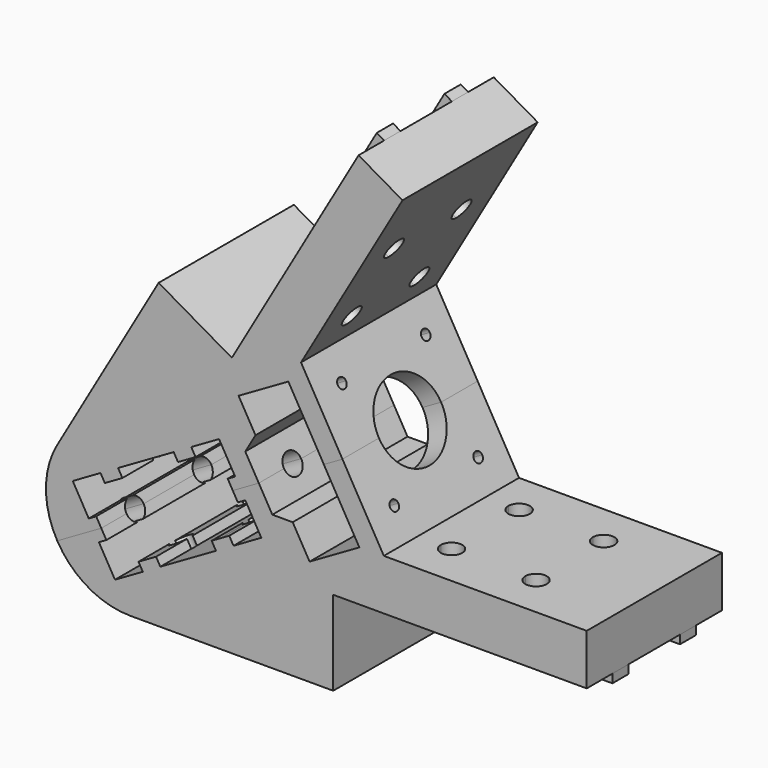
from build123d import *
from build123d import SkipClean  # not in build123d's __all__

# Parameters (mm, degrees)
F1_DEPTH  = 50
F3_DEPTH  = 50
F4_W      = 6
F4_H      = 75
F5_DEPTH  = 2.54
F7_DEPTH  = 78.4977147554
F8_W      = 53.81
F8_H      = 3.175
F13_W     = 6.35
F13_H     = 6.35
F17_DEPTH = 6.35
F19_DEPTH = 50.0010001
F22_W     = 3.175
F22_H     = 8.0837567297
F22_H_2   = 12.5575134595
F22_H_3   = 6.35


with BuildPart() as f1:
    # F0 (on Front) → F1 (new body)
    with BuildSketch(Plane.XZ):
        with BuildLine():
            Line((80.4903810568, 109.4134295109), (67.5, 116.9134295109))
            Line((67.5, 116.9134295109), (30, 51.9615242271))
            Line((30, 51.9615242271), (8.3493649054, 64.4615242271))
            Line((8.3493649054, 64.4615242271), (-21.6506350946, 12.5))
            ThreePointArc((-21.6506350946, 12.5), (-25, 0), (-21.6506350946, -12.5))
            Line((-21.6506350946, -12.5), (-10.8253175473, -6.25))
            Line((-10.8253175473, -6.25), (-17.0753175473, 4.5753175473))
            Line((-17.0753175473, 4.5753175473), (-6.25, 10.8253175473))
            Line((-6.25, 10.8253175473), (26.2259526419, 29.5753175473))
            Line((26.2259526419, 29.5753175473), (32.4759526419, 18.75))
            Line((32.4759526419, 18.75), (37.9752139559, 21.925))
            Line((37.9752139559, 21.925), (33.9770633418, 28.85))
            Line((33.9770633418, 28.85), (46.8086730745, 51.075))
            Line((46.8086730745, 51.075), (50.4748472839, 57.425))
            Line((50.4748472839, 57.425), (80.4903810568, 109.4134295109))
        make_face()
        Polygon((62.7218898691, 36.2125), (50.4748472839, 57.425), (46.8086730745, 51.075), (57.2226285551, 33.0375), align=None)
    extrude(amount=F1_DEPTH)

    # F2 (on face) → F3 (join, through all)
    with BuildSketch(Plane(origin=(0, 0, 0), x_dir=(-1, 0, 0), z_dir=(0, 1, 0))):
        Polygon((-15.4006350946, 23.3253175473), (-17.998711306, 24.8253175473), (-19.268711306, 22.6256130217), (-16.6706350946, 21.1256130217), align=None)
        Polygon((-12.8025588833, 21.8253175473), (-15.4006350946, 23.3253175473), (-16.6706350946, 21.1256130217), (-14.0725588833, 19.6256130217), align=None)
        Polygon((-28.7762481163, 20.0780762114), (-30.9759526419, 21.3480762114), (-32.4759526419, 18.75), (-30.2762481163, 17.48), align=None)
        Polygon((10.8253175473, -6.25), (12.3253175473, -3.6519237886), (10.1256130217, -2.3819237886), (8.6256130217, -4.98), align=None)
        Polygon((6.25, 10.8253175473), (3.6519237886, 12.3253175473), (2.3819237886, 10.1256130217), (4.98, 8.6256130217), align=None)
        Polygon((8.8480762114, 9.3253175473), (6.25, 10.8253175473), (4.98, 8.6256130217), (7.5780762114, 7.1256130217), align=None)
    extrude(amount=-F3_DEPTH)

    # F4 (on face) → F5 (join)
    with BuildSketch(Plane(origin=(0, 0, 0), x_dir=(0, -1, 0), z_dir=(-0.8660254038, 0, 0.5))):
        with Locations((12.5, 97.5)):
            Rectangle(F4_W, F4_H)
        with Locations((37.5, 97.5)):
            Rectangle(F4_W, F4_H)
    extrude(amount=F5_DEPTH)

    # F6 (on face) → F7 (cut, through all)
    with BuildSketch(Plane(origin=(-2.1997045256, 0, 1.27), x_dir=(0, -1, 0), z_dir=(-0.8660254038, 0, 0.5))):
        with BuildLine():
            ThreePointArc((12.5, 88.175), (9.325, 85), (12.5, 81.825))
            Line((12.5, 81.825), (12.5, 85))
            Line((12.5, 85), (12.5, 88.175))
        make_face()
        with BuildLine():
            ThreePointArc((12.5, 113.175), (9.325, 110), (12.5, 106.825))
            Line((12.5, 106.825), (12.5, 110))
            Line((12.5, 110), (12.5, 113.175))
        make_face()
        with BuildLine():
            Line((12.5, 110), (12.5, 106.825))
            ThreePointArc((12.5, 106.825), (14.7450640303, 107.7549359697), (15.675, 110))
            ThreePointArc((15.675, 110), (14.7450640303, 112.2450640303), (12.5, 113.175))
            Line((12.5, 113.175), (12.5, 110))
        make_face()
        with BuildLine():
            Line((12.5, 85), (12.5, 81.825))
            ThreePointArc((12.5, 81.825), (14.7450640303, 82.7549359697), (15.675, 85))
            ThreePointArc((15.675, 85), (14.7450640303, 87.2450640303), (12.5, 88.175))
            Line((12.5, 88.175), (12.5, 85))
        make_face()
        with BuildLine():
            ThreePointArc((37.5, 88.175), (34.325, 85), (37.5, 81.825))
            Line((37.5, 81.825), (37.5, 85))
            Line((37.5, 85), (37.5, 88.175))
        make_face()
        with BuildLine():
            ThreePointArc((37.5, 113.175), (34.325, 110), (37.5, 106.825))
            Line((37.5, 106.825), (37.5, 110))
            Line((37.5, 110), (37.5, 113.175))
        make_face()
        with BuildLine():
            Line((37.5, 110), (37.5, 106.825))
            ThreePointArc((37.5, 106.825), (39.7450640303, 107.7549359697), (40.675, 110))
            ThreePointArc((40.675, 110), (39.7450640303, 112.2450640303), (37.5, 113.175))
            Line((37.5, 113.175), (37.5, 110))
        make_face()
        with BuildLine():
            Line((37.5, 85), (37.5, 81.825))
            ThreePointArc((37.5, 81.825), (39.7450640303, 82.7549359697), (40.675, 85))
            ThreePointArc((40.675, 85), (39.7450640303, 87.2450640303), (37.5, 88.175))
            Line((37.5, 88.175), (37.5, 85))
        make_face()
    extrude(amount=-F7_DEPTH, mode=Mode.SUBTRACT)

    # F8 (on face) → F9 (revolve, cut)
    with BuildSketch(Plane(origin=(0, 0, 0), x_dir=(0.8660254038, 0, 0.5), z_dir=(0.5, 0, -0.8660254038))):
        Polygon((-9.96, 9.325), (-9.96, 12.5), (-25, 12.5), (-25, 6.15), (-21.825, 6.15), (-21.825, 9.325), align=None)
        with Locations((16.945, 10.9125)):
            Rectangle(F8_W, F8_H)
    revolve(axis=Axis((-15.1381240582, -12.5, -8.74), (-0.8660254038, 0, -0.5)), mode=Mode.SUBTRACT)

    # F8 (on face) → F10 (revolve, cut)
    with BuildSketch(Plane(origin=(0, 0, 0), x_dir=(0.8660254038, 0, 0.5), z_dir=(0.5, 0, -0.8660254038))):
        Polygon((-21.825, 34.325), (-9.96, 34.325), (-9.96, 37.5), (-25, 37.5), (-25, 31.15), (-21.825, 31.15), align=None)
        with Locations((16.945, 35.9125)):
            Rectangle(F8_W, F8_H)
    revolve(axis=Axis((-15.1381240582, -37.5, -8.74), (-0.8660254038, 0, -0.5)), mode=Mode.SUBTRACT)

    # F13 (on face) → F14 (revolve, cut)
    with BuildSketch(Plane(origin=(21.6506350946, 0, 12.5), x_dir=(0, 1, 0), z_dir=(0.8660254038, 0, 0.5))):
        with Locations((-9.325, 46.4762701892)):
            Rectangle(F13_W, F13_H)
        Polygon((-12.5, 9.96), (-9.325, 9.96), (-9.325, 36.9512701892), (-6.15, 36.9512701892), (-6.15, 43.3012701892), (-12.5, 43.3012701892), align=None)
    revolve(axis=Axis((8.3353175473, -12.5, 35.5628065108), (-0.5, 0, 0.8660254038)), mode=Mode.SUBTRACT)

    # F13 (on face) → F15 (revolve, cut)
    with BuildSketch(Plane(origin=(21.6506350946, 0, 12.5), x_dir=(0, 1, 0), z_dir=(0.8660254038, 0, 0.5))):
        with Locations((-34.325, 46.4762701892)):
            Rectangle(F13_W, F13_H)
        Polygon((-37.5, 9.96), (-34.325, 9.96), (-34.325, 36.9512701892), (-31.15, 36.9512701892), (-31.15, 43.3012701892), (-37.5, 43.3012701892), align=None)
    revolve(axis=Axis((6.7478175473, -37.5, 38.3124371679), (-0.5, 0, 0.8660254038)), mode=Mode.SUBTRACT)

    # F16 (on face) → F17 (cut, through all)
    with BuildSketch(Plane(origin=(62.7218898691, 0, 36.2125), x_dir=(0, 1, 0), z_dir=(0.8660254038, 0, 0.5))):
        with BuildLine():
            ThreePointArc((-8, 15.5), (-9.5, 17), (-11, 15.5))
            Line((-11, 15.5), (-9.5, 15.5))
            Line((-9.5, 15.5), (-9.5, 14))
            ThreePointArc((-9.5, 14), (-8.4393398282, 14.4393398282), (-8, 15.5))
        make_face()
        with BuildLine():
            Line((-9.5, 15.5), (-11, 15.5))
            ThreePointArc((-11, 15.5), (-10.5606601718, 14.4393398282), (-9.5, 14))
            Line((-9.5, 14), (-9.5, 15.5))
        make_face()
        with BuildLine():
            ThreePointArc((-40.5, 14), (-39.4393398282, 14.4393398282), (-39, 15.5))
            Line((-39, 15.5), (-40.5, 15.5))
            Line((-40.5, 15.5), (-40.5, 14))
        make_face()
        with BuildLine():
            Line((-40.5, 15.5), (-39, 15.5))
            ThreePointArc((-39, 15.5), (-41.5606601718, 16.5606601718), (-40.5, 14))
            Line((-40.5, 14), (-40.5, 15.5))
        make_face()
        with BuildLine():
            ThreePointArc((-13.5, 0), (-25, 11.5), (-36.5, 0))
            Line((-36.5, 0), (-13.5, 0))
        make_face()
    extrude(amount=-F17_DEPTH, mode=Mode.SUBTRACT)

    # F18 (on face) → F19 (cut, through all)
    with BuildSketch(Plane.XZ.offset(50)):
        Polygon((46.7226285551, 51.2240334795), (32.0001966907, 42.7240334795), (36.9937184983, 34.075), (46.8086730745, 51.075), align=None)
    extrude(amount=-F19_DEPTH, mode=Mode.SUBTRACT)

    # F22 (on face) → F23 (revolve, cut)
    with BuildSketch(Plane(origin=(0, 0, 0), x_dir=(0, 1, 0), z_dir=(0.8660254038, 0, 0.5))):
        Polygon((-40.675, 28.8675134595), (-40.675, 36.9512701892), (-37.5, 36.9512701892), (-37.5, 41.5675134595), (-43.85, 41.5675134595), (-43.85, 28.8675134595), align=None)
        with Locations((-39.0875, 32.9093918244)):
            Rectangle(F22_W, F22_H)
        with Locations((-39.0875, 16.2387567297)):
            Rectangle(F22_W, F22_H_2)
        with Locations((-39.0875, 25.6925134595)):
            Rectangle(F22_W, F22_H_3)
        with Locations((-42.2625, 25.6925134595)):
            Rectangle(F22_W, F22_H_3)
    revolve(axis=Axis((-12.8818783649, -37.5, 22.3120678249), (0.5, 0, -0.8660254038)), mode=Mode.SUBTRACT)

    # F22 (on face) → F24 (revolve, cut)
    with BuildSketch(Plane(origin=(0, 0, 0), x_dir=(0, 1, 0), z_dir=(0.8660254038, 0, 0.5))):
        with Locations((-17.2625, 25.6925134595)):
            Rectangle(F22_W, F22_H_3)
        with Locations((-14.0875, 25.6925134595)):
            Rectangle(F22_W, F22_H_3)
        with Locations((-14.0875, 16.2387567297)):
            Rectangle(F22_W, F22_H_2)
        Polygon((-18.85, 41.5675134595), (-18.85, 28.8675134595), (-15.675, 28.8675134595), (-15.675, 36.9512701892), (-12.5, 36.9512701892), (-12.5, 41.5675134595), align=None)
        with Locations((-14.0875, 32.9093918244)):
            Rectangle(F22_W, F22_H)
    revolve(axis=Axis((-12.8818783649, -12.5, 22.3120678249), (0.5, 0, -0.8660254038)), mode=Mode.SUBTRACT)

    # F25: F1 across face


with BuildPart() as f1_1:
    add(f1.part, clean=False)
    with SkipClean():  # cleaning this boolean's faces spoils the solid; the shape is the same uncleaned
        add(f1.part.mirror(Plane(origin=(-14.740242609, -45.575638949, -8.5102830382), x_dir=(0, 1, 0), z_dir=(0.5, 0, -0.8660254038))), clean=False)


solid = f1_1.part
